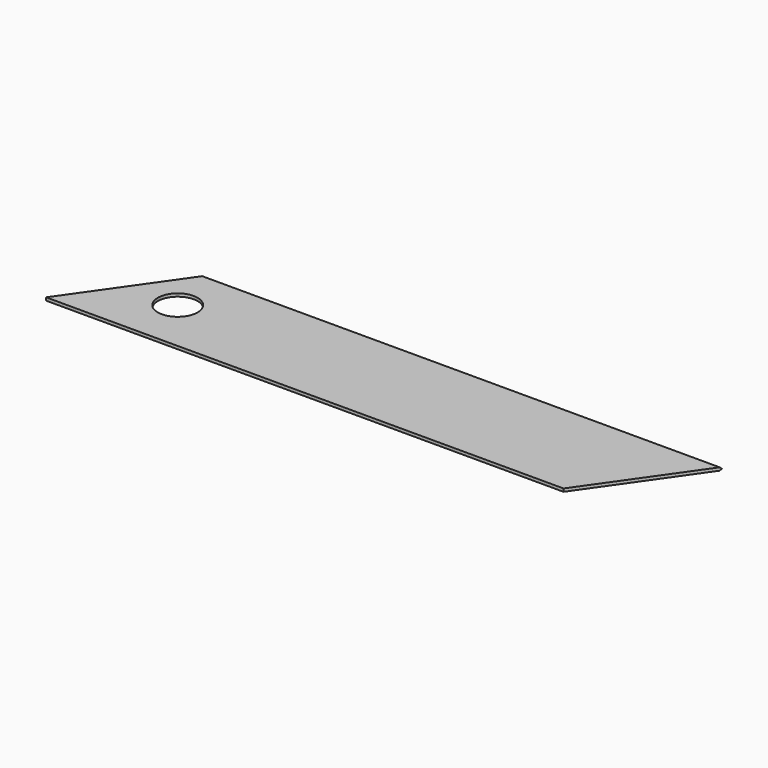
from build123d import *

# Parameters (mm, degrees)
F0_R        = 3.341537713
F1_DEPTH    = 0.5
F2_T1_DEPTH = 89.571682988


# Not quite as in the source:
# - a fillet or chamfer that OpenCascade refuses, or shapes differently, is made with other operations: its cross-section is extruded or revolved along the edge and cut away or added


with BuildPart() as f1:
    # F0 (on Top) → F1 (new body)
    with BuildSketch(Plane.XY):
        Polygon((16.2269707607, 8.9300729632), (3.6232350729, -9.0699270368), (90.6232350729, -9.0699270368), (103.2269707607, 8.9300729632), align=None)
        with Locations((18.4976458549, 0)):
            Circle(F0_R, mode=Mode.SUBTRACT)
    extrude(amount=F1_DEPTH)

    # F2: chamfer of 0.5 on 2 edges, made by hand

    # F2_s2 → F2_t1 (cut)
    with BuildSketch(Plane.YZ.offset(14.9411292667)):
        Polygon((8.9300729632, 0), (8.4300729632, 0.5), (8.9300729632, 0.5), align=None)
        Polygon((8.9300729632, 0.5), (8.4300729632, 0), (8.9300729632, 0), align=None)
    extrude(amount=F2_T1_DEPTH, mode=Mode.SUBTRACT)


solid = f1.part
